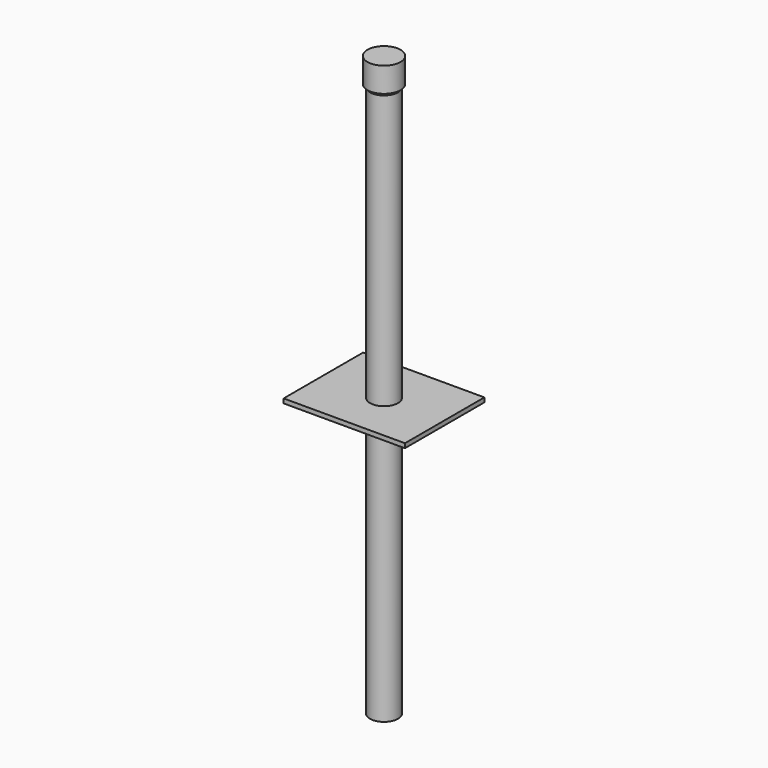
from build123d import *

# Parameters (mm, degrees)
F0_W          = 220
F0_H          = 180
F1_DEPTH      = 4
F1_DEPTH_BACK = 4
F2_R          = 5
F3_DEPTH      = 50
F3_DEPTH_BACK = 50
F4_R          = 25.5
F4_R_2        = 24
F5_DEPTH      = 500
F5_DEPTH_BACK = 500
F6_R          = 30
F6_R_2        = 25.5
F6_R_3        = 24
F7_DEPTH      = 50
F8_SIZE       = 5


with BuildPart() as f1:
    # F0 (on Top) → F1 (new body, two sides)
    with BuildSketch(Plane.XY) as f1_sk:
        Rectangle(F0_W, F0_H)
    extrude(amount=F1_DEPTH)
    extrude(f1_sk.sketch, amount=-F1_DEPTH_BACK)


with BuildPart() as f3:
    # F2 (on Top) → F3 (new body, two sides)
    with BuildSketch(Plane.XY) as f3_sk:
        Circle(F2_R)
    extrude(amount=F3_DEPTH)
    extrude(f3_sk.sketch, amount=-F3_DEPTH_BACK)


with BuildPart() as f5:
    # F4 (on Top) → F5 (new body, two sides)
    with BuildSketch(Plane.XY) as f5_sk:
        Circle(F4_R)
        Circle(F4_R_2, mode=Mode.SUBTRACT)
    extrude(amount=F5_DEPTH)
    extrude(f5_sk.sketch, amount=-F5_DEPTH_BACK)


with BuildPart() as f7:
    # F6 (on face) → F7 (new body)
    with BuildSketch(Plane.XY.offset(500)):
        Circle(F6_R)
        Circle(F6_R_2, mode=Mode.SUBTRACT)
        Circle(F6_R_2)
        Circle(F6_R_3, mode=Mode.SUBTRACT)
        Circle(F6_R_3)
    extrude(amount=F7_DEPTH)

    # F8
    f8_edges = [f7.edges().sort_by_distance(p)[0] for p in [
        (-30, 0, 500),
    ]]
    chamfer(f8_edges, length=F8_SIZE)


with BuildPart() as f10:
    # F9 (on Top) → F10 (revolve)
    with BuildSketch(Plane.XY):
        with BuildLine():
            Line((0, 0), (0, 23.5))
            ThreePointArc((0, 23.5), (-23.5, 0), (0, -23.5))
            Line((0, -23.5), (0, 0))
        make_face()
    revolve(axis=Axis((0, 0, 0), (0, -1, 0)))


solid = Compound([f1.part, f3.part, f5.part, f7.part, f10.part])
